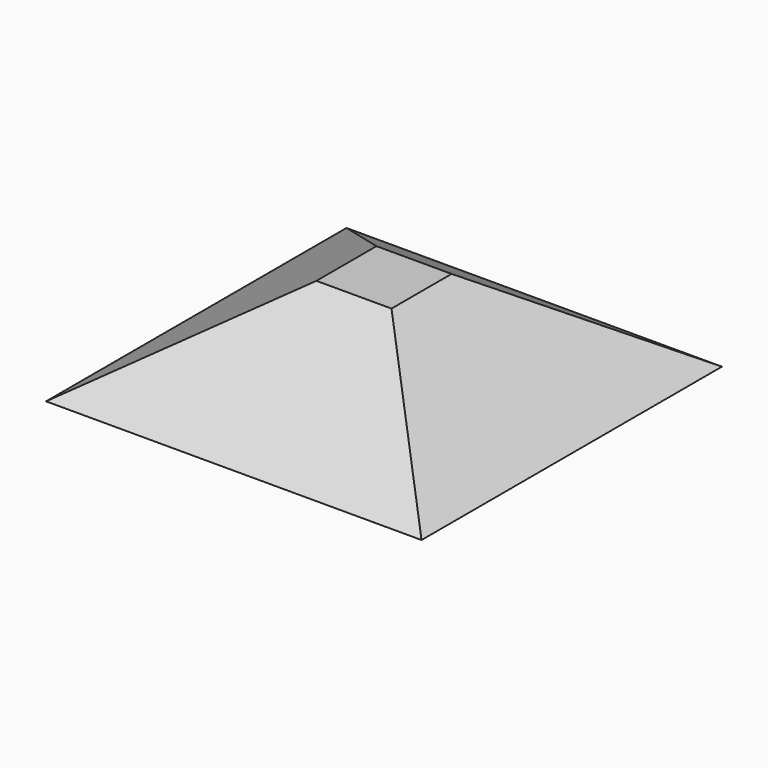
from build123d import *

# Parameters (mm, degrees)
F0_W     = 25.4
F0_H     = 25.4
F1_DEPTH = 6.35
F2_SIZE2 = 10.15999
F2_SIZE  = 6.34999


# Not quite as in the source:
# - a fillet or chamfer is up to 0.001 mm smaller than in the source, because OpenCascade refuses the exact size


with BuildPart() as f1:
    # F0 (on Top) → F1 (new body)
    with BuildSketch(Plane.XY):
        with Locations((-6.5350332297, 3.7000408258)):
            Rectangle(F0_W, F0_H)
    extrude(amount=F1_DEPTH)

    # F2 (size 6.35 and 10.16 in the source; OpenCascade refuses exactly that, so slightly less here)
    f2_edges = [f1.edges().sort_by_distance(p)[0] for p in [
        (-6.535033, 16.400041, 6.35),
        (-19.235033, 3.700041, 6.35),
        (-6.535033, -8.999959, 6.35),
        (6.164967, 3.700041, 6.35),
    ]]
    chamfer(f2_edges, length=F2_SIZE, length2=F2_SIZE2)


solid = f1.part
